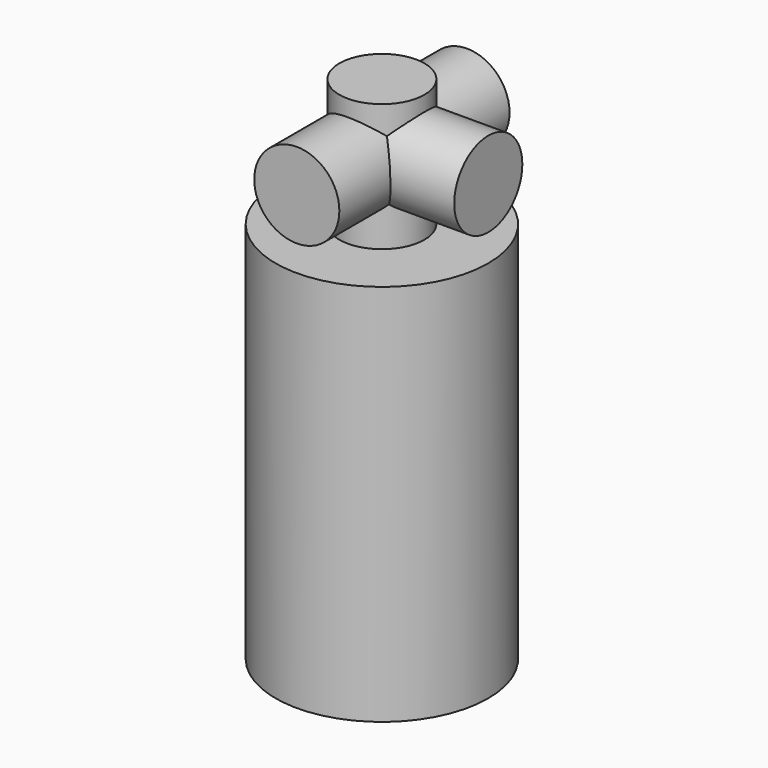
from build123d import *

# Parameters (mm, degrees)
F0_R     = 31.75
F1_DEPTH = 114.3
F2_R     = 12.7
F3_DEPTH = 38.1
F4_R     = 12.7
F5_DEPTH = 31.75
F6_R     = 12.7
F7_DEPTH = 31.75


# Not quite as in the source:
# - a pattern or mirror of a feature is missing from the dataset's text; its kind, count and spacing are read off the source's solid


with BuildPart() as f1:
    # F0 (on Top) → F1 (new body)
    with BuildSketch(Plane.XY):
        Circle(F0_R)
    extrude(amount=F1_DEPTH)

    # F2 (on face) → F3 (join)
    with BuildSketch(Plane.XY.offset(114.3)):
        Circle(F2_R)
    extrude(amount=F3_DEPTH)

    # F4 (on Front) → F5 (join)
    with BuildSketch(Plane.XZ):
        with Locations((0, 134.8038613796)):
            Circle(F4_R)
    f5 = extrude(amount=F5_DEPTH)

    # F5_copies: F5 across plane
    add(f5.mirror(Plane.ZX))


with BuildPart() as f7:
    # F6 (on Right) → F7 (new body)
    with BuildSketch(Plane.YZ):
        with Locations((0, 135.1637542248)):
            Circle(F6_R)
    extrude(amount=F7_DEPTH)


solid = Compound([f1.part, f7.part])
